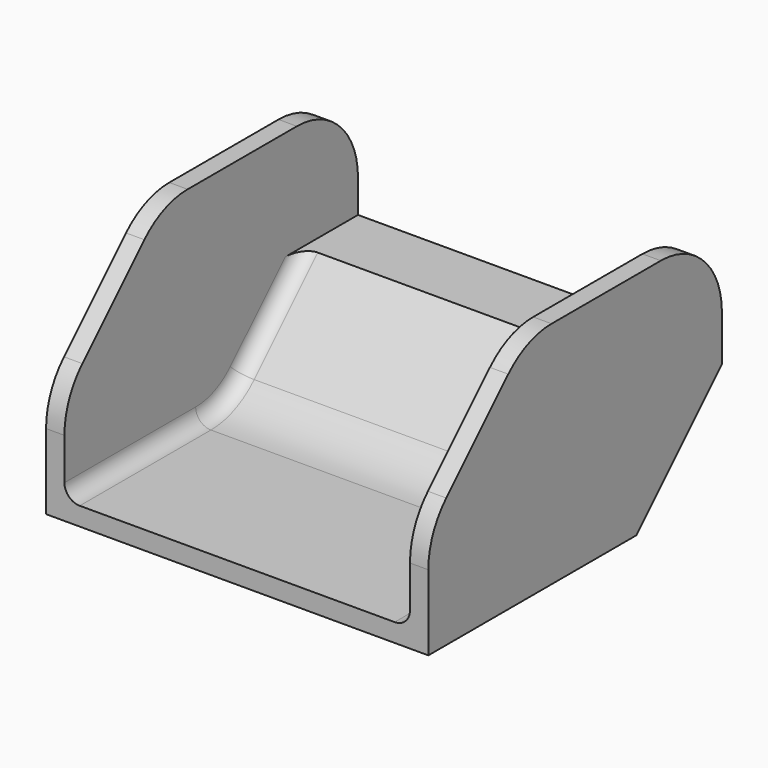
from build123d import *

# Parameters (mm, degrees)
F0_W        = 25
F0_H        = 24
F1_DEPTH    = 15
F2_T        = -1.2
F3_DEPTH    = 25
F4_W        = 22.6
F4_H        = 7.1360613033
F5_DEPTH    = 25
F6_T4_DEPTH = 22.6
F7_R        = 5
F8_SIZE     = 8
F9_R        = 5
F10_R       = 1
F11_SIZE    = 7


# Not quite as in the source:
# - a fillet or chamfer that OpenCascade refuses, or shapes differently, is made with other operations: its cross-section is extruded or revolved along the edge and cut away or added


with BuildPart() as f1:
    # F0 (on Top) → F1 (new body)
    with BuildSketch(Plane.XY):
        with Locations((-29.1051699208, 12)):
            Rectangle(F0_W, F0_H)
    extrude(amount=F1_DEPTH)

    # F2
    f2_openings = [f1.faces().sort_by_distance(p)[0] for p in [
        (-29.10517, 12, 15),
    ]]
    offset(amount=F2_T, openings=f2_openings)

    # F3 (cut): a face of the model
    f3_faces = [f1.faces().sort_by_distance(p)[0] for p in [
        (-29.1051699208, 1.2, 8.1),
    ]]
    extrude(f3_faces, amount=-F3_DEPTH, mode=Mode.SUBTRACT)

    # F4 (on face) → F5 (cut)
    with BuildSketch(Plane.XZ.offset(-22.8)):
        with Locations((-29.1051699208, 11.4319693483)):
            Rectangle(F4_W, F4_H)
    extrude(amount=-F5_DEPTH, mode=Mode.SUBTRACT)

    # F6: chamfer of 10 on 1 edges, made by hand


with BuildPart() as f6_tool2:
    # F6_s3 → F6_t4 (new body)
    with BuildSketch(Plane.YZ.offset(-17.8051699208)):
        Polygon((22.8, 11.2), (12.8, 1.2), (22.8, 1.2), align=None)
    extrude(amount=-F6_T4_DEPTH)

    split(bisect_by=Plane.XY.offset(7.8639386967), keep=Keep.BOTTOM)


with BuildPart() as f1_1:
    add(f1.part)

    # F6_t1: union F6_tool2
    add(f6_tool2.part)

    # F7
    f7_edges = [f1_1.edges().sort_by_distance(p)[0] for p in [
        (-29.10517, 12.8, 1.2),
        (-17.20517, 24, 15),
        (-41.00517, 24, 15),
    ]]
    fillet(f7_edges, radius=F7_R)

    # F8
    f8_edges = [f1_1.edges().sort_by_distance(p)[0] for p in [
        (-41.00517, 0, 15),
        (-17.20517, 0, 15),
    ]]
    chamfer(f8_edges, length=F8_SIZE)

    # F9
    f9_edges = [f1_1.edges().sort_by_distance(p)[0] for p in [
        (-41.00517, 8, 15),
        (-41.00517, 0, 7),
        (-17.20517, 0, 7),
        (-17.20517, 8, 15),
    ]]
    fillet(f9_edges, radius=F9_R)

    # F10
    f10_edges = [f1_1.edges().sort_by_distance(p)[0] for p in [
        (-40.40517, 5.364466, 1.2),
        (-17.80517, 5.364466, 1.2),
        (-17.80517, 12.642349, 1.580602),
        (-17.80517, 16.864202, 5.264202),
        (-40.40517, 16.864202, 5.264202),
        (-40.40517, 12.642349, 1.580602),
    ]]
    fillet(f10_edges, radius=F10_R)

    # F11
    f11_edges = [f1_1.edges().sort_by_distance(p)[0] for p in [
        (-29.10517, 24, 0),
    ]]
    chamfer(f11_edges, length=F11_SIZE)


solid = f1_1.part
